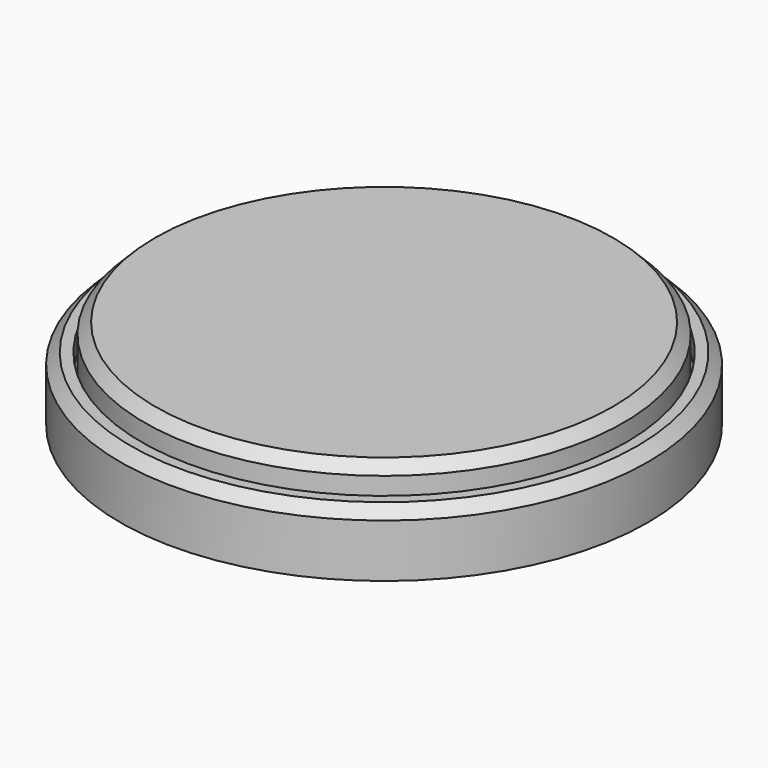
from build123d import *

# Parameters (mm, degrees)
F0_W     = 20
F0_H     = 2
F2_SIZE  = 1
F3_R     = 24.8
F3_R_2   = 22.8
F3_R_3   = 22.5
F4_DEPTH = 4
F5_DEPTH = 2
F6_SIZE  = 1


with BuildPart() as f1:
    # F0 (on Front) → F1 (revolve)
    with BuildSketch(Plane.XZ):
        Polygon((-22.5, 0), (0, 0), (0, 2.5), (-20, 2.5), (-20, 4.5), (-22.5, 4.5), (-22.5, 2.5), align=None)
        with Locations((-10, 3.5)):
            Rectangle(F0_W, F0_H)
    revolve(axis=Axis((0, 0, 1.25), (0, 0, 1)))

    # F2
    f2_edges = [f1.edges().sort_by_distance(p)[0] for p in [
        (22.5, 0, 4.5),
    ]]
    chamfer(f2_edges, length=F2_SIZE)


with BuildPart() as f4:
    # F3 (on face) → F4 (new body)
    with BuildSketch(Plane(origin=(0, 0, 0), x_dir=(1, 0, 0), z_dir=(0, 0, -1))):
        Circle(F3_R)
        Circle(F3_R_2, mode=Mode.SUBTRACT)
        Circle(F3_R_2)
        Circle(F3_R_3, mode=Mode.SUBTRACT)
        Circle(F3_R_3)
    extrude(amount=F4_DEPTH)

    # F3 (on face) → F5 (join)
    with BuildSketch(Plane(origin=(0, 0, 0), x_dir=(1, 0, 0), z_dir=(0, 0, -1))):
        Circle(F3_R)
        Circle(F3_R_2, mode=Mode.SUBTRACT)
    extrude(amount=-F5_DEPTH)

    # F6
    f6_edges = [f4.edges().sort_by_distance(p)[0] for p in [
        (-24.8, 0, 2),
    ]]
    chamfer(f6_edges, length=F6_SIZE)


solid = Compound([f1.part, f4.part])
